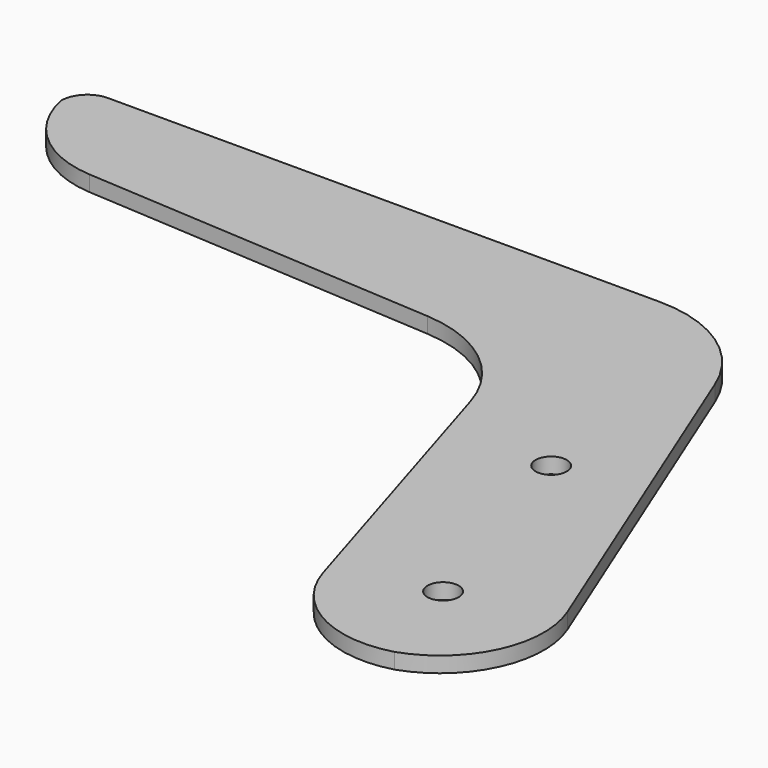
from build123d import *

# Parameters (mm, degrees)
F0_R        = 3
F1_DEPTH    = 3
F2_R        = 5
F3_T1_DEPTH = 103
F3_T3_DEPTH = 112.1308501069
F4_T1_DEPTH = 95.1083829874
F5_R        = 25


# Not quite as in the source:
# - a fillet or chamfer that OpenCascade refuses, or shapes differently, is made with other operations: its cross-section is extruded or revolved along the edge and cut away or added


with BuildPart() as f1:
    # F0 (on Top) → F1 (new body)
    with BuildSketch(Plane.XY):
        Polygon((43.4865237426, -107.6329232161), (0, 0), (-128, 0), (-128, -20), (-23.896152608, -26.506490462), (4.5464630903, -119.5380944954), align=None)
        with Locations((16.5764476545, -93.9006322304)):
            Circle(F0_R, mode=Mode.SUBTRACT)
        with Locations((3.7120926467, -51.8232229681)):
            Circle(F0_R, mode=Mode.SUBTRACT)
    extrude(amount=F1_DEPTH)

    # F2
    f2_edges = [f1.edges().sort_by_distance(p)[0] for p in [
        (-128, 0, 1.5),
    ]]
    fillet(f2_edges, radius=F2_R)

    # F3: fillet of radius 20 on 2 edges, made by hand

    # F3_s2 → F3_t1 (cut)
    with BuildSketch(Plane.XY.offset(-50)):
        with BuildLine():
            ThreePointArc((23.6725582096, -113.6906604009), (8.4356928594, -112.2235171388), (-1.3009710041, -100.4119993761))
            Line((-1.3009710041, -100.4119993761), (4.5464630903, -119.5380944954))
            Line((4.5464630903, -119.5380944954), (23.6725582096, -113.6906604009))
        make_face()
    extrude(amount=F3_T1_DEPTH, mode=Mode.SUBTRACT)

    # F3_s4 → F3_t3 (cut)
    with BuildSketch(Plane.XY.offset(-54.5654250535)):
        with BuildLine():
            ThreePointArc((35.3102965436, -87.3960507653), (34.8183251392, -103.4984045697), (22.6140535467, -114.0142777528))
            Line((22.6140535467, -114.0142777528), (43.4865237426, -107.6329232161))
            Line((43.4865237426, -107.6329232161), (35.3102965436, -87.3960507653))
        make_face()
    extrude(amount=F3_T3_DEPTH, mode=Mode.SUBTRACT)

    # F4: fillet of radius 20 on 1 edges, made by hand

    # F4_s2 → F4_t1 (cut)
    with BuildSketch(Plane.XY.offset(-46.0541914937)):
        with BuildLine():
            ThreePointArc((-109.6141981719, -21.1491126143), (-121.5651855194, -16.2146440508), (-128, -5))
            Line((-128, -5), (-128.392667351, -5.0762387791))
            ThreePointArc((-128.392667351, -5.0762387791), (-128.4, -12.5), (-128.4, -20))
            Line((-128.4, -20), (-128.0249513145, -20.3992210314))
            Line((-128.0249513145, -20.3992210314), (-109.6391494864, -21.5483336456))
            Line((-109.6391494864, -21.5483336456), (-109.6141981719, -21.1491126143))
        make_face()
    extrude(amount=F4_T1_DEPTH, mode=Mode.SUBTRACT)

    # F5
    f5_edges = [f1.edges().sort_by_distance(p)[0] for p in [
        (0, 0, 1.5),
        (-23.896153, -26.50649, 1.5),
    ]]
    fillet(f5_edges, radius=F5_R)


solid = f1.part
